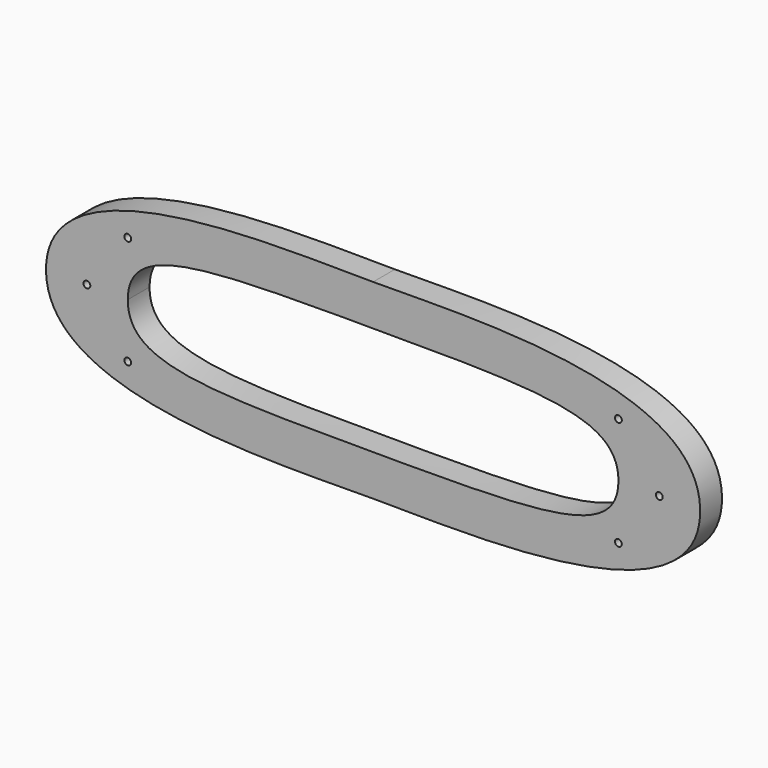
from build123d import *

# Parameters (mm, degrees)
F0_R     = 3.175
F1_DEPTH = 25.4


# Not quite as in the source:
# - ends of sketch curves that miss each other by under 0.0002 mm in the source are joined


with BuildPart() as f1:
    # F0 (on Front) → F1 (new body)
    with BuildSketch(Plane.XZ):
        with BuildLine():
            add(Edge.make_bspline(
                [(-304.8, 5.2081e-06), (-304.8, 101.6000008473), (-80.1557193555, 88.5515600587), (-1.5676e-06, 88.9)],
                knots=[0, 0, 0, 0, 317.4999970368, 317.4999970368, 317.4999970368, 317.4999970368], degree=3))
            add(Edge.make_bspline(
                [(-304.8, 5.2081e-06), (-304.8, -101.6000008473), (-80.1557193555, -88.5515600587), (-1.5676e-06, -88.9)],
                knots=[0, 0, 0, 0, 317.4999970368, 317.4999970368, 317.4999970368, 317.4999970368], degree=3))
            add(Edge.make_bspline(
                [(304.8, -5.2081e-06), (304.8, -101.6000008473), (80.1557193555, -88.5515600587), (-1.5676e-06, -88.9)],
                knots=[0, 0, 0, 0, 317.4999970368, 317.4999970368, 317.4999970368, 317.4999970368], degree=3))
            add(Edge.make_bspline(
                [(304.8, -5.2081e-06), (304.8, 101.6000008473), (80.1557193555, 88.5515600587), (-1.5676e-06, 88.9)],
                knots=[0, 0, 0, 0, 317.4999970368, 317.4999970368, 317.4999970368, 317.4999970368], degree=3))
        make_face()
        with Locations((-228.5999996275, -50.8)):
            Circle(F0_R, mode=Mode.SUBTRACT)
        with Locations((228.5999996275, -50.8)):
            Circle(F0_R, mode=Mode.SUBTRACT)
        with Locations((-266.7, 0)):
            Circle(F0_R, mode=Mode.SUBTRACT)
        with Locations((-228.5999996275, 50.8)):
            Circle(F0_R, mode=Mode.SUBTRACT)
        with BuildLine():
            add(Edge.make_bspline(
                [(-228.6, 0), (-228.5999996275, -50.8), (-155.7715911424, -50.8), (8.682e-07, -50.8)],
                knots=[0, 0, 0, 0, 234.1764300628, 234.1764300628, 234.1764300628, 234.1764300628], degree=3))
            add(Edge.make_bspline(
                [(-228.6, 0), (-228.5999996275, 50.8), (-155.7715911424, 50.8), (8.682e-07, 50.8)],
                knots=[0, 0, 0, 0, 234.1764300628, 234.1764300628, 234.1764300628, 234.1764300628], degree=3))
            add(Edge.make_bspline(
                [(228.6, 0), (228.5999996275, 50.8), (155.7715911424, 50.8), (8.682e-07, 50.8)],
                knots=[0, 0, 0, 0, 234.1764300628, 234.1764300628, 234.1764300628, 234.1764300628], degree=3))
            add(Edge.make_bspline(
                [(228.6, 0), (228.5999996275, -50.8), (155.7715911424, -50.8), (8.682e-07, -50.8)],
                knots=[0, 0, 0, 0, 234.1764300628, 234.1764300628, 234.1764300628, 234.1764300628], degree=3))
        make_face(mode=Mode.SUBTRACT)
        with Locations((266.7, 0)):
            Circle(F0_R, mode=Mode.SUBTRACT)
        with Locations((228.5999996275, 50.8)):
            Circle(F0_R, mode=Mode.SUBTRACT)
    extrude(amount=F1_DEPTH)


solid = f1.part
